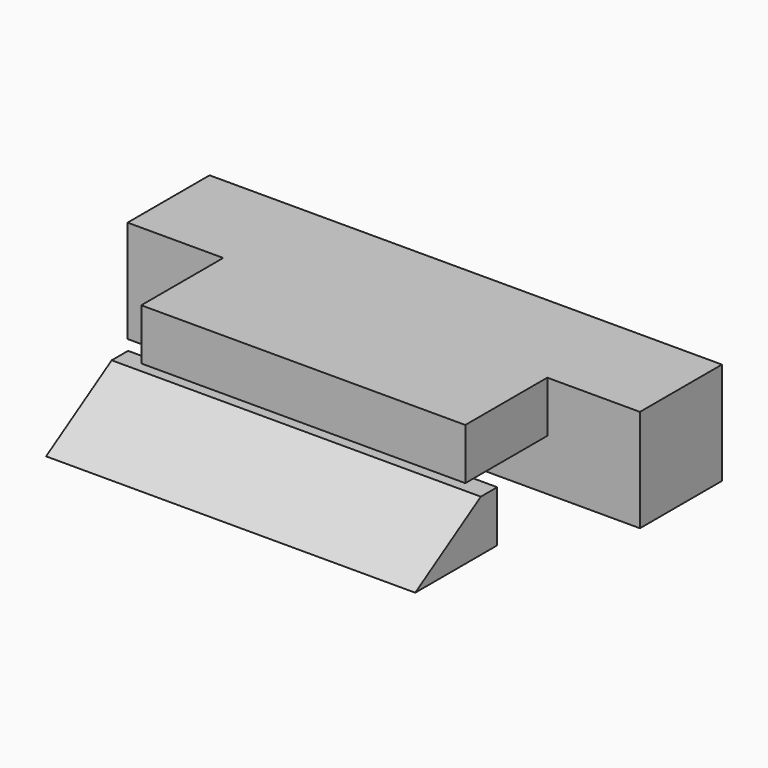
from build123d import *

# Parameters (mm, degrees)
F0_W     = 6.3244109941
F0_H     = 2
F1_DEPTH = 1
F2_DEPTH = 1
F3_W     = 7.2049933622
F3_H     = 2
F4_DEPTH = 1
F5_SIZE2 = 0.99999
F5_SIZE  = 1.59999


# Not quite as in the source:
# - a fillet or chamfer is up to 0.001 mm smaller than in the source, because OpenCascade refuses the exact size


with BuildPart() as f1:
    # F0 (on Top) → F1 (new body)
    with BuildSketch(Plane.XY):
        Polygon((-13.5638297198, 2), (-23.5638297198, 2), (-23.5638297198, 0), (-21.6967508232, 0), (-15.3723398291, 0), (-13.5638297198, 0), align=None)
        with Locations((-18.5345453261, -1)):
            Rectangle(F0_W, F0_H)
    extrude(amount=F1_DEPTH)

    # F0 (on Top) → F2 (join)
    with BuildSketch(Plane.XY):
        Polygon((-13.5638297198, 2), (-23.5638297198, 2), (-23.5638297198, 0), (-21.6967508232, 0), (-15.3723398291, 0), (-13.5638297198, 0), align=None)
    extrude(amount=-F2_DEPTH)

    # F3 (on face) → F4 (join)
    with BuildSketch(Plane(origin=(0, 0, -1), x_dir=(1, 0, 0), z_dir=(0, 0, -1))):
        with Locations((-18.5119810809, 2.8)):
            Rectangle(F3_W, F3_H)
    extrude(amount=-F4_DEPTH)

    # F5 (size 1.6 and 1 in the source; OpenCascade refuses exactly that, so slightly less here)
    f5_edges = [f1.edges().sort_by_distance(p)[0] for p in [
        (-18.511981, -3.8, 0),
    ]]
    f5_side = f1.faces().sort_by_distance((-18.50981, -2.886602, 0))[0]
    chamfer(f5_edges, length=F5_SIZE, length2=F5_SIZE2, reference=f5_side)


solid = f1.part
